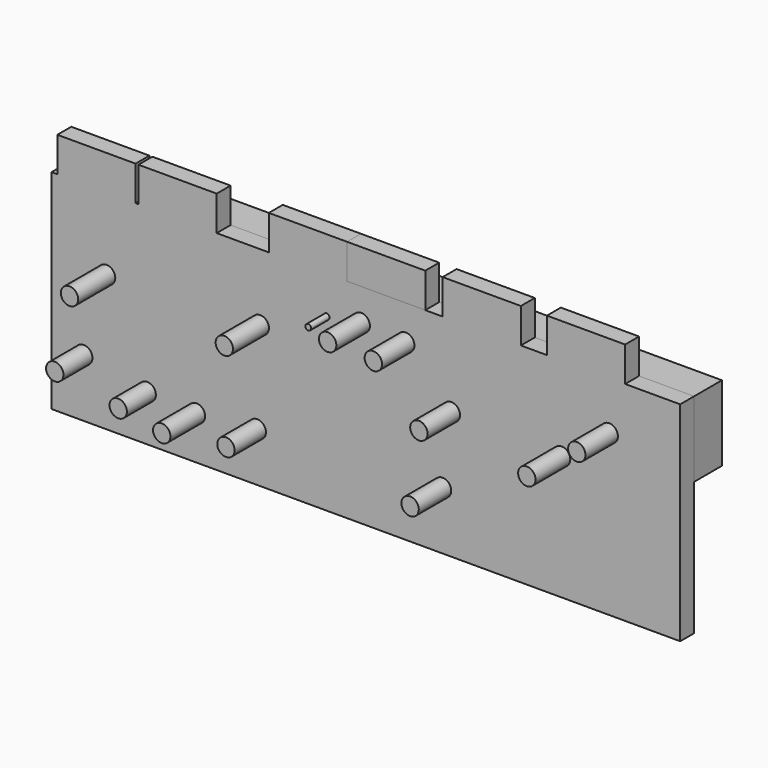
from build123d import *

# Parameters (mm, degrees)
F0_W      = 688.975
F0_H      = 228.6
F1_DEPTH  = 19.05
F2_W      = 688.975
F2_H      = 82.55
F3_DEPTH  = 38.1
F4_R      = 9.525
F5_DEPTH  = 50.8
F6_DEPTH  = 49.2125
F7_DEPTH  = 46.0375
F8_DEPTH  = 44.45
F9_DEPTH  = 44.45
F10_DEPTH = 39.6875
F11_DEPTH = 39.6875
F12_DEPTH = 47.625
F13_DEPTH = 42.8625
F14_DEPTH = 44.45
F15_DEPTH = 47.625
F16_DEPTH = 44.45
F4_R_2    = 3.175
F17_DEPTH = 25.4
F18_W     = 85.725
F18_H     = 19.05
F19_DEPTH = 38.1
F20_DEPTH = 38.1
F21_DEPTH = 38.1
F22_DEPTH = 38.1


with BuildPart() as f1:
    # F0 (on Front) → F1 (new body)
    with BuildSketch(Plane.XZ):
        Rectangle(F0_W, F0_H)
    extrude(amount=F1_DEPTH)

    # F4 (on face) → F5 (join)
    with BuildSketch(Plane.XZ.offset(19.05)):
        with Locations((-284.177719027, 34.921354228)):
            Circle(F4_R)
    extrude(amount=F5_DEPTH)

    # F4 (on face) → F6 (join)
    with BuildSketch(Plane.XZ.offset(19.05)):
        with Locations((-115.7773256969, 41.2260214307)):
            Circle(F4_R)
    extrude(amount=F6_DEPTH)

    # F4 (on face) → F7 (join)
    with BuildSketch(Plane.XZ.offset(19.05)):
        with Locations((-5.0731406292, 79.4205398983)):
            Circle(F4_R)
    extrude(amount=F7_DEPTH)

    # F4 (on face) → F8 (join)
    with BuildSketch(Plane.XZ.offset(19.05)):
        with Locations((43.7131791432, 76.3541009185)):
            Circle(F4_R)
    extrude(amount=F8_DEPTH)

    # F4 (on face) → F9 (join)
    with BuildSketch(Plane.XZ.offset(19.05)):
        with Locations((266.7021014949, 61.2707650235)):
            Circle(F4_R)
    extrude(amount=F9_DEPTH)

    # F4 (on face) → F10 (join)
    with BuildSketch(Plane.XZ.offset(19.05)):
        with Locations((-309.2386653451, -50.5142142372)):
            Circle(F4_R)
    extrude(amount=F10_DEPTH)

    # F4 (on face) → F11 (join)
    with BuildSketch(Plane.XZ.offset(19.05)):
        with Locations((-239.704221487, -63.5)):
            Circle(F4_R)
    extrude(amount=F11_DEPTH)

    # F4 (on face) → F12 (join)
    with BuildSketch(Plane.XZ.offset(19.05)):
        with Locations((-185.6680512428, -66.6236951947)):
            Circle(F4_R)
    extrude(amount=F12_DEPTH)

    # F4 (on face) → F13 (join)
    with BuildSketch(Plane.XZ.offset(19.05)):
        with Locations((-119.0625, -60.3054687381)):
            Circle(F4_R)
    extrude(amount=F13_DEPTH)

    # F4 (on face) → F14 (join)
    with BuildSketch(Plane.XZ.offset(19.05)):
        with Locations((93.636199832, 25.4305675626)):
            Circle(F4_R)
    extrude(amount=F14_DEPTH)

    # F4 (on face) → F15 (join)
    with BuildSketch(Plane.XZ.offset(19.05)):
        with Locations((214.4906967878, 21.935204044)):
            Circle(F4_R)
    extrude(amount=F15_DEPTH)

    # F4 (on face) → F16 (join)
    with BuildSketch(Plane.XZ.offset(19.05)):
        with Locations((84.0205475688, -50.6887696683)):
            Circle(F4_R)
    extrude(amount=F16_DEPTH)

    # F4 (on face) → F17 (join)
    with BuildSketch(Plane.XZ.offset(19.05)):
        with Locations((-42.8788997233, 73.0070248246)):
            Circle(F4_R_2)
    extrude(amount=F17_DEPTH)

    # F18 (on face) → F19 (join)
    with BuildSketch(Plane.XY.offset(114.3)):
        with Locations((-295.275, -9.525)):
            Rectangle(F18_W, F18_H)
    extrude(amount=F19_DEPTH)

    # F18 (on face) → F20 (join)
    with BuildSketch(Plane.XY.offset(114.3)):
        with Locations((-206.375, -9.525)):
            Rectangle(F18_W, F18_H)
        with Locations((-63.5, -9.525)):
            Rectangle(F18_W, F18_H)
    extrude(amount=F20_DEPTH)

    # F18 (on face) → F22 (join)
    with BuildSketch(Plane.XY.offset(114.3)):
        with Locations((127, -9.525)):
            Rectangle(F18_W, F18_H)
        with Locations((241.3, -9.525)):
            Rectangle(F18_W, F18_H)
    extrude(amount=F22_DEPTH)


with BuildPart() as f3:
    # F2 (on face) → F3 (new body)
    with BuildSketch(Plane(origin=(0, 0, 0), x_dir=(-1, 0, 0), z_dir=(0, 1, 0))):
        with Locations((0, 73.025)):
            Rectangle(F2_W, F2_H)
    extrude(amount=F3_DEPTH)


with BuildPart() as f21:
    # F18 (on face) → F21 (new body)
    with BuildSketch(Plane.XY.offset(114.3)):
        with Locations((22.225, -9.525)):
            Rectangle(F18_W, F18_H)
    extrude(amount=F21_DEPTH)


solid = Compound([f1.part, f3.part, f21.part])
